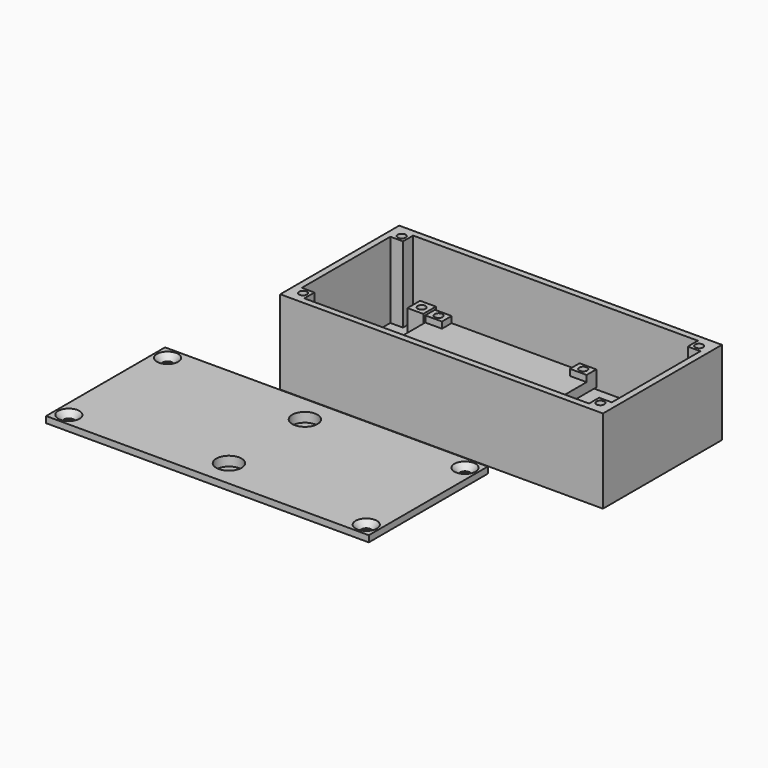
from build123d import *

# Parameters (mm, degrees)
F0_W             = 102
F0_H             = 47
F1_DEPTH         = 26.5
F2_W             = 98
F2_H             = 43
F3_DEPTH         = 24
F4_W             = 64.5
F4_H             = 13.8
F5_DEPTH         = 26.501
F6_W             = 5
F6_H             = 5
F7_DEPTH         = 8.9
F12_D            = 2.5
F12_DEPTH        = 6.5
F12_TIP          = 0.7510757738
F12_ON_F9_D      = 2.5
F12_ON_F9_DEPTH  = 6.5
F12_ON_F9_TIP    = 0.7510757738
F12_ON_F11_D     = 2.5
F12_ON_F11_DEPTH = 6.5
F12_ON_F11_TIP   = 0.7510757738
F12_ON_F10_D     = 2.5
F12_ON_F10_DEPTH = 6.5
F12_ON_F10_TIP   = 0.7510757738
F13_W            = 4
F13_H            = 4
F14_DEPTH        = 24
F16_D            = 2.5
F16_DEPTH        = 9.5
F16_TIP          = 0.7510757738
F17_W            = 102
F17_H            = 47
F18_DEPTH        = 2
F20_D            = 3.15
F20_CSINK_D      = 6.72
F20_CSINK_ANGLE  = 90
F21_W            = 87.28
F21_H            = 39
F22_DEPTH        = 4
F23_R            = 4
F24_DEPTH        = 3
F25_W            = 51
F25_H            = 3
F26_DEPTH        = 22.86
F27_W            = 5.279949
F27_H            = 3.81
F27_H_2          = 3.855
F27_W_2          = 5.280051
F28_DEPTH        = 2
F33_D            = 2.54
F33_DEPTH        = 5
F33_TIP          = 0.7630929862
F33_ON_F30_D     = 2.54
F33_ON_F30_DEPTH = 5
F33_ON_F30_TIP   = 0.7630929862
F33_ON_F32_D     = 2.54
F33_ON_F32_DEPTH = 5
F33_ON_F32_TIP   = 0.7630929862
F33_ON_F31_D     = 2.54
F33_ON_F31_DEPTH = 5
F33_ON_F31_TIP   = 0.7630929862


# Not quite as in the source:
# - a feature names something its author has since deleted; it is built from what else it names


with BuildPart() as f1:
    # F0 (on Top) → F1 (new body)
    with BuildSketch(Plane.XY):
        Rectangle(F0_W, F0_H)
    extrude(amount=F1_DEPTH)

    # F2 (on face) → F3 (cut)
    with BuildSketch(Plane.XY.offset(26.5)):
        Rectangle(F2_W, F2_H)
    extrude(amount=-F3_DEPTH, mode=Mode.SUBTRACT)

    # F4 (on face) → F5 (cut, through all)
    with BuildSketch(Plane(origin=(0, 0, 0), x_dir=(1, 0, 0), z_dir=(0, 0, -1))):
        Rectangle(F4_W, F4_H)
    extrude(amount=-F5_DEPTH, mode=Mode.SUBTRACT)

    # F6 (on face) → F7 (join)
    with BuildSketch(Plane.XY.offset(2.5)):
        with Locations((-37.5, 15.5)):
            Rectangle(F6_W, F6_H)
        with Locations((-37.5, -15.5)):
            Rectangle(F6_W, F6_H)
        with Locations((37.5, -15.5)):
            Rectangle(F6_W, F6_H)
        with Locations((37.5, 15.5)):
            Rectangle(F6_W, F6_H)
    extrude(amount=F7_DEPTH)

    # F12
    with Locations(Plane.XY.offset(11.4)):
        with Locations((-37.5, 15.5)):
            Hole(F12_D / 2, depth=F12_DEPTH)
            with Locations((0, 0, -(F12_DEPTH + F12_TIP / 2))):  # 118° drill point
                Cone(0, F12_D / 2, F12_TIP, mode=Mode.SUBTRACT)

    # F12 on F9
    with Locations(Plane.XY.offset(11.4)):
        with Locations((-37.5, -15.5)):
            Hole(F12_ON_F9_D / 2, depth=F12_ON_F9_DEPTH)
            with Locations((0, 0, -(F12_ON_F9_DEPTH + F12_ON_F9_TIP / 2))):  # 118° drill point
                Cone(0, F12_ON_F9_D / 2, F12_ON_F9_TIP, mode=Mode.SUBTRACT)

    # F12 on F11
    with Locations(Plane.XY.offset(11.4)):
        with Locations((37.5, -15.5)):
            Hole(F12_ON_F11_D / 2, depth=F12_ON_F11_DEPTH)
            with Locations((0, 0, -(F12_ON_F11_DEPTH + F12_ON_F11_TIP / 2))):  # 118° drill point
                Cone(0, F12_ON_F11_D / 2, F12_ON_F11_TIP, mode=Mode.SUBTRACT)

    # F12 on F10
    with Locations(Plane.XY.offset(11.4)):
        with Locations((37.5, 15.5)):
            Hole(F12_ON_F10_D / 2, depth=F12_ON_F10_DEPTH)
            with Locations((0, 0, -(F12_ON_F10_DEPTH + F12_ON_F10_TIP / 2))):  # 118° drill point
                Cone(0, F12_ON_F10_D / 2, F12_ON_F10_TIP, mode=Mode.SUBTRACT)

    # F13 (on face) → F14 (join)
    with BuildSketch(Plane.XY.offset(2.5)):
        with Locations((-47, -19.5)):
            Rectangle(F13_W, F13_H)
        with Locations((-47, 19.5)):
            Rectangle(F13_W, F13_H)
        with Locations((47, 19.5)):
            Rectangle(F13_W, F13_H)
        with Locations((47, -19.5)):
            Rectangle(F13_W, F13_H)
    extrude(amount=F14_DEPTH)

    # F16
    with Locations(Plane.XY.offset(26.5)):
        with Locations((-47, -19.5), (-47, 19.5), (47, 19.5), (47, -19.5)):
            Hole(F16_D / 2, depth=F16_DEPTH)
            with Locations((0, 0, -(F16_DEPTH + F16_TIP / 2))):  # 118° drill point
                Cone(0, F16_D / 2, F16_TIP, mode=Mode.SUBTRACT)

    # F25 (on face) → F26 (join)
    with BuildSketch(Plane(origin=(0, -21.5, 0), x_dir=(-1, 0, 0), z_dir=(0, 1, 0))):
        with Locations((-3.5, 18)):
            Rectangle(F25_W, F25_H)
    extrude(amount=F26_DEPTH)

    # F27 (on face) → F28 (join)
    with BuildSketch(Plane.XY.offset(19.5)):
        with Locations((26.3600255, -0.545)):
            Rectangle(F27_W, F27_H)
        with Locations((26.3600255, -19.5725)):
            Rectangle(F27_W, F27_H_2)
        with Locations((-19.3599745, -19.595)):
            Rectangle(F27_W_2, F27_H)
        with Locations((-19.3599745, -0.545)):
            Rectangle(F27_W_2, F27_H)
    extrude(amount=F28_DEPTH)

    # F33
    with Locations(Plane.XY.offset(21.5)):
        with Locations((26.360051, -0.5000000002)):
            Hole(F33_D / 2, depth=F33_DEPTH)
            with Locations((0, 0, -(F33_DEPTH + F33_TIP / 2))):  # 118° drill point
                Cone(0, F33_D / 2, F33_TIP, mode=Mode.SUBTRACT)

    # F33 on F30
    with Locations(Plane.XY.offset(21.5)):
        with Locations((26.3599551176, -19.5500000013)):
            Hole(F33_ON_F30_D / 2, depth=F33_ON_F30_DEPTH)
            with Locations((0, 0, -(F33_ON_F30_DEPTH + F33_ON_F30_TIP / 2))):  # 118° drill point
                Cone(0, F33_ON_F30_D / 2, F33_ON_F30_TIP, mode=Mode.SUBTRACT)

    # F33 on F32
    with Locations(Plane.XY.offset(21.5)):
        with Locations((-19.36, -0.5000000002)):
            Hole(F33_ON_F32_D / 2, depth=F33_ON_F32_DEPTH)
            with Locations((0, 0, -(F33_ON_F32_DEPTH + F33_ON_F32_TIP / 2))):  # 118° drill point
                Cone(0, F33_ON_F32_D / 2, F33_ON_F32_TIP, mode=Mode.SUBTRACT)

    # F33 on F31
    with Locations(Plane.XY.offset(21.5)):
        with Locations((-19.3603835499, -19.6399999571)):
            Hole(F33_ON_F31_D / 2, depth=F33_ON_F31_DEPTH)
            with Locations((0, 0, -(F33_ON_F31_DEPTH + F33_ON_F31_TIP / 2))):  # 118° drill point
                Cone(0, F33_ON_F31_D / 2, F33_ON_F31_TIP, mode=Mode.SUBTRACT)


with BuildPart() as f18:
    # F17 (on Top) → F18 (new body)
    with BuildSketch(Plane.XY):
        with Locations((-33.8762627295, -50.1713193953)):
            Rectangle(F17_W, F17_H)
    extrude(amount=F18_DEPTH)

    # F20 (through all)
    with Locations(Plane.XY.offset(2)):
        with Locations((-80.8762627295, -30.6713193953), (-80.8762627295, -69.6713193953), (13.1237372705, -69.6713193953), (13.1237372705, -30.6713193953)):
            CounterSinkHole(F20_D / 2, F20_CSINK_D / 2, counter_sink_angle=F20_CSINK_ANGLE)

    # F21 (on face) → F22 (join)
    with BuildSketch(Plane.XY.offset(2)):
        with Locations((-33.8762627295, -50.1713193953)):
            Rectangle(F21_W, F21_H)
    extrude(amount=-F22_DEPTH)

    # F23 (on face) → F24 (cut)
    with BuildSketch(Plane.XY.offset(2)):
        with Locations((-33.8762627295, -35.1713193953)):
            Circle(F23_R)
        with Locations((-33.8762627295, -65.1713193953)):
            Circle(F23_R)
    extrude(amount=-F24_DEPTH, mode=Mode.SUBTRACT)


solid = Compound([f1.part, f18.part])
